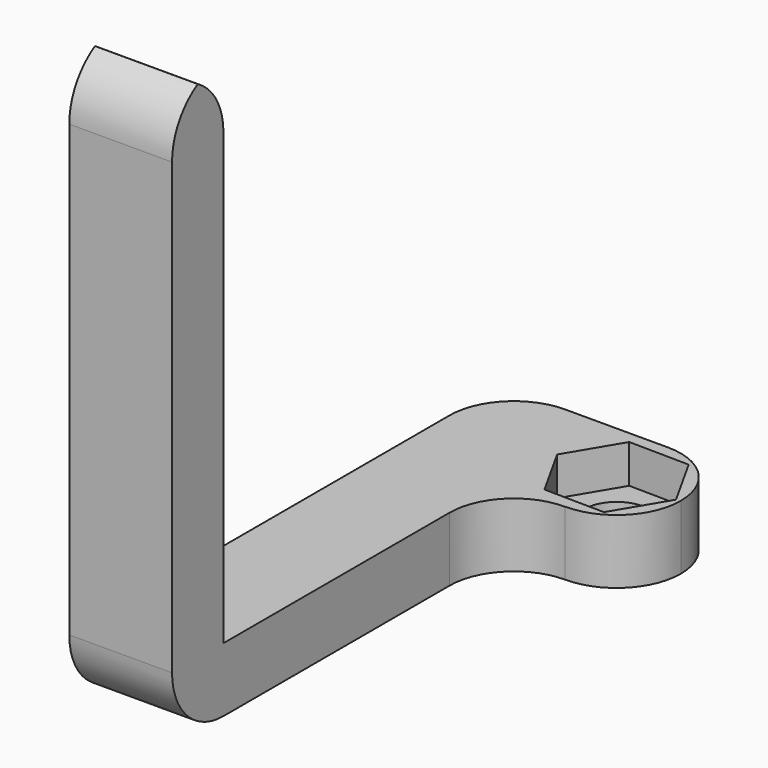
from build123d import *

# Parameters (mm, degrees)
F0_W        = 8
F0_H        = 5
F1_DEPTH    = 45
F0_R        = 2.5
F2_DEPTH    = 5
F3_DEPTH    = 10
F4_DEPTH    = 2
F5_T1_DEPTH = 5
F5_T3_DEPTH = 30
F5_T5_DEPTH = 33


# Not quite as in the source:
# - a fillet or chamfer that OpenCascade refuses, or shapes differently, is made with other operations: its cross-section is extruded or revolved along the edge and cut away or added


with BuildPart() as f1:
    # F0 (on Top) → F1 (new body)
    with BuildSketch(Plane.XY):
        with Locations((-5, -21)):
            Rectangle(F0_W, F0_H)
    extrude(amount=F1_DEPTH)

    # F0 (on Top) → F2 (join)
    with BuildSketch(Plane.XY):
        Polygon((9, 18.5), (-9, 18.5), (-9, -18.5), (-1, -18.5), (-1, 8.5), (9, 8.5), align=None)
        Polygon((1.6027649533, 9.4804546863), (-0.6796458767, 13.5662937924), (1.71758917, 17.5858391061), (6.3972350467, 17.5195453137), (8.6796458767, 13.4337062076), (6.28241083, 9.4141608939), align=None, mode=Mode.SUBTRACT)
        Polygon((1.71758917, 17.5858391061), (-0.6796458767, 13.5662937924), (1.6027649533, 9.4804546863), (6.28241083, 9.4141608939), (8.6796458767, 13.4337062076), (6.3972350467, 17.5195453137), align=None)
        with Locations((4, 13.5)):
            Circle(F0_R, mode=Mode.SUBTRACT)
    extrude(amount=F2_DEPTH)

    # F0 (on Top) → F3 (cut)
    with BuildSketch(Plane.XY):
        Polygon((1.71758917, 17.5858391061), (-0.6796458767, 13.5662937924), (1.6027649533, 9.4804546863), (6.28241083, 9.4141608939), (8.6796458767, 13.4337062076), (6.3972350467, 17.5195453137), align=None)
        with Locations((4, 13.5)):
            Circle(F0_R, mode=Mode.SUBTRACT)
    extrude(amount=F3_DEPTH, mode=Mode.SUBTRACT)

    # F0 (on Top) → F4 (join)
    with BuildSketch(Plane.XY):
        Polygon((1.71758917, 17.5858391061), (-0.6796458767, 13.5662937924), (1.6027649533, 9.4804546863), (6.28241083, 9.4141608939), (8.6796458767, 13.4337062076), (6.3972350467, 17.5195453137), align=None)
        with Locations((4, 13.5)):
            Circle(F0_R, mode=Mode.SUBTRACT)
    extrude(amount=F4_DEPTH)

    # F5: fillet of radius 5 on 7 edges, made by hand

    # F5_s2 → F5_t1 (join)
    with BuildSketch(Plane.XY):
        with BuildLine():
            ThreePointArc((-1, 3.5), (0.4644660941, 7.0355339059), (4, 8.5))
            Line((4, 8.5), (-1, 8.5))
            Line((-1, 8.5), (-1, 3.5))
        make_face()
    extrude(amount=F5_T1_DEPTH)

    # F5_s4 → F5_t3 (cut)
    with BuildSketch(Plane.XY.offset(-12.5)):
        with BuildLine():
            ThreePointArc((-9, 13.5), (-7.5355339059, 17.0355339059), (-4, 18.5))
            Line((-4, 18.5), (-9, 18.5))
            Line((-9, 18.5), (-9, 13.5))
        make_face()
        with BuildLine():
            ThreePointArc((4, 18.5), (7.5355339059, 17.0355339059), (9, 13.5))
            Line((9, 13.5), (9, 18.5))
            Line((9, 18.5), (4, 18.5))
        make_face()
        with BuildLine():
            ThreePointArc((9, 13.5), (7.5355339059, 9.9644660941), (4, 8.5))
            Line((4, 8.5), (9, 8.5))
            Line((9, 8.5), (9, 13.5))
        make_face()
    extrude(amount=F5_T3_DEPTH, mode=Mode.SUBTRACT)

    # F5_s6 → F5_t5 (cut)
    with BuildSketch(Plane.YZ.offset(-21.5)):
        with BuildLine():
            ThreePointArc((-23.5, 5), (-22.0355339059, 1.4644660941), (-18.5, 0))
            Line((-18.5, 0), (-23.5, 0))
            Line((-23.5, 0), (-23.5, 5))
        make_face()
        with BuildLine():
            ThreePointArc((-18.5, 45), (-22.0355339059, 43.5355339059), (-23.5, 40))
            Line((-23.5, 40), (-23.5, 45))
            Line((-23.5, 45), (-18.5, 45))
        make_face()
        with BuildLine():
            ThreePointArc((-18.5, 40), (-19.9644660941, 43.5355339059), (-23.5, 45))
            Line((-23.5, 45), (-18.5, 45))
            Line((-18.5, 45), (-18.5, 40))
        make_face()
    extrude(amount=F5_T5_DEPTH, mode=Mode.SUBTRACT)


solid = f1.part
